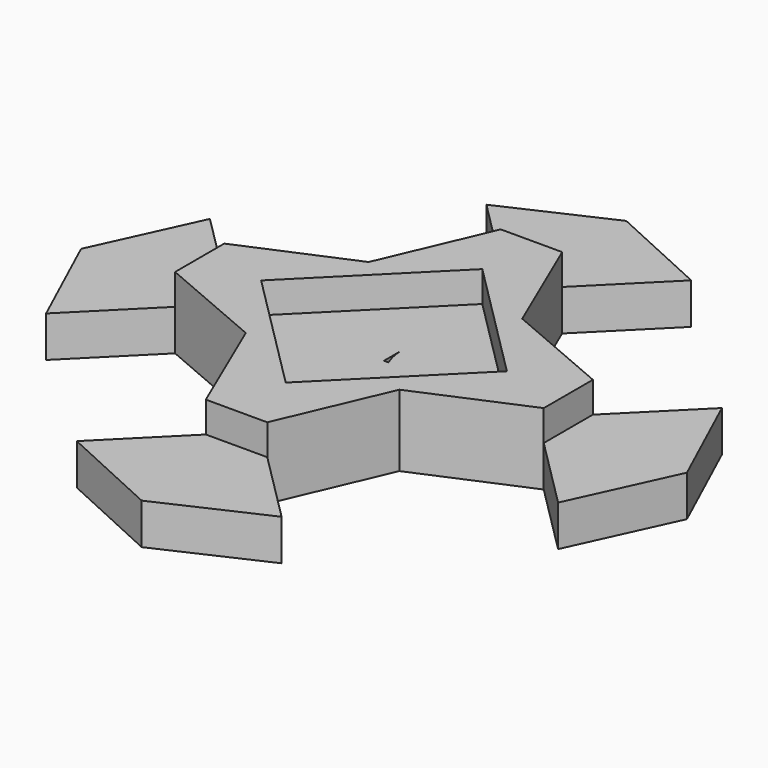
from build123d import *

# Parameters (mm, degrees)
F1_DEPTH = 10.16
F3_DEPTH = 7.62


# Not quite as in the source:
# - a feature names something its author has since deleted; it is built from what else it names


with BuildPart() as f1:
    # F0 (on Top) → F1 (new body)
    with BuildSketch(Plane.XY):
        Polygon((-19.05, 19.05), (0, 0), (0, 5.2605122421), (0, 38.1), align=None)
        with BuildLine():
            Line((1.1407175417, 0), (0, 0))
            Line((0, 0), (0, -38.1))
            Line((0, -38.1), (19.05, -19.05))
            Line((19.05, -19.05), (3.7197438789, -3.7197438789))
            ThreePointArc((3.7197438789, -3.7197438789), (2.263176494, -1.9756963719), (1.1407175417, 0))
        make_face()
        Polygon((-19.05, -19.05), (0, 0), (-38.1, 0), align=None)
        Polygon((-38.1, 0), (0, 0), (-19.05, 19.05), align=None)
        Polygon((0, -38.1), (0, 0), (-19.05, -19.05), align=None)
        with BuildLine():
            Line((0, 38.1), (0, 5.2605122421))
            ThreePointArc((0, 5.2605122421), (0.2032791438, 2.9973357481), (0.8066091092, 0.8066091092))
            Line((0.8066091092, 0.8066091092), (19.05, 19.05))
            Line((19.05, 19.05), (0, 38.1))
        make_face()
        with BuildLine():
            ThreePointArc((0.8066091092, 0.8066091092), (0.9667299371, 0.4004326511), (1.1407175417, 0))
            Line((1.1407175417, 0), (38.1, 0))
            Line((38.1, 0), (19.05, 19.05))
            Line((19.05, 19.05), (0.8066091092, 0.8066091092))
        make_face()
        with BuildLine():
            Line((38.1, 0), (1.1407175417, 0))
            ThreePointArc((1.1407175417, 0), (2.263176494, -1.9756963719), (3.7197438789, -3.7197438789))
            Line((3.7197438789, -3.7197438789), (19.05, -19.05))
            Line((19.05, -19.05), (38.1, 0))
        make_face()
        Polygon((7.62, -45.72), (0, -38.1), (0, -63.5), align=None)
        Polygon((-7.62, -45.72), (0, -38.1), (-19.05, -19.05), align=None)
        Polygon((19.05, -19.05), (0, -38.1), (7.62, -45.72), align=None)
        Polygon((0, -63.5), (0, -38.1), (-7.62, -45.72), align=None)
        Polygon((-45.72, -7.62), (-38.1, 0), (-63.5, 0), align=None)
        Polygon((-45.72, 7.62), (-38.1, 0), (-19.05, 19.05), align=None)
        Polygon((-63.5, 0), (-38.1, 0), (-45.72, 7.62), align=None)
        Polygon((-19.05, -19.05), (-38.1, 0), (-45.72, -7.62), align=None)
        Polygon((-7.62, 45.72), (-19.05, 19.05), (0, 38.1), align=None)
        Polygon((-7.62, 45.72), (0, 38.1), (0, 63.5), align=None)
        Polygon((7.62, 45.72), (0, 38.1), (19.05, 19.05), align=None)
        Polygon((0, 63.5), (0, 38.1), (7.62, 45.72), align=None)
        Polygon((45.72, 7.62), (38.1, 0), (63.5, 0), align=None)
        Polygon((45.72, -7.62), (38.1, 0), (19.05, -19.05), align=None)
        Polygon((19.05, 19.05), (38.1, 0), (45.72, 7.62), align=None)
        Polygon((63.5, 0), (38.1, 0), (45.72, -7.62), align=None)
        Polygon((7.62, -45.72), (0, -63.5), (-7.62, -45.72), (-25.4, -63.5), (0, -75.1397422652), (25.4, -63.5), align=None)
        Polygon((-45.72, -7.62), (-63.5, 0), (-45.72, 7.62), (-63.5, 25.4), (-75.1397422652, 0), (-63.5, -25.4), align=None)
        Polygon((-25.4, 63.5), (-7.62, 45.72), (0, 63.5), (7.62, 45.72), (25.4, 63.5), (0, 75.1238912344), align=None)
        Polygon((45.72, 7.62), (63.5, 0), (45.72, -7.62), (63.5, -25.4), (75.1397422652, 0), (63.5, 25.4), align=None)
    extrude(amount=F1_DEPTH)

    # F2 (on face) → F3 (join)
    with BuildSketch(Plane.XY.offset(10.16)):
        Polygon((-19.05, 19.05), (-45.72, 7.62), (-45.72, -7.62), (-19.05, -19.05), (-7.62, -45.72), (7.62, -45.72), (19.05, -19.05), (45.72, -7.62), (45.72, 7.62), (19.05, 19.05), (7.62, 45.72), (-7.62, 45.72), align=None)
        Polygon((0, -30.48), (-30.48, 0), (0, 30.48), (30.48, 0), align=None, mode=Mode.SUBTRACT)
    extrude(amount=F3_DEPTH)


solid = f1.part
